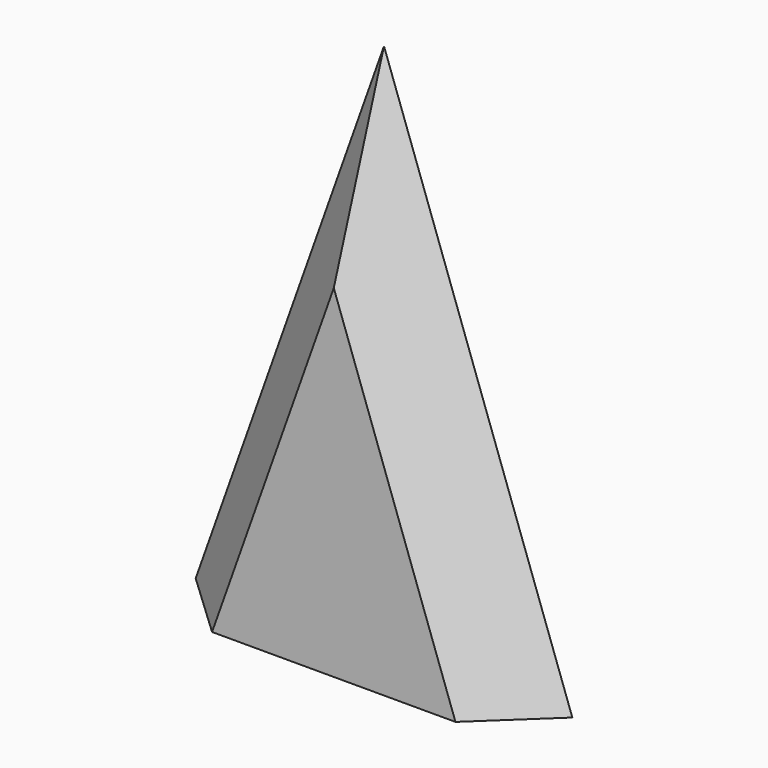
from build123d import *

# Parameters (mm, degrees)
F1_DEPTH      = 2.54
F1_DEPTH_BACK = 2.54
F2_R          = 1.905
F3_DEPTH      = 5.08
F4_SIZE       = 2.53999


# Not quite as in the source:
# - a fillet or chamfer is up to 0.001 mm smaller than in the source, because OpenCascade refuses the exact size


with BuildPart() as f1:
    # F0 (on Front) → F1 (new body, two sides)
    with BuildSketch(Plane.XZ) as f1_sk:
        Polygon((0, 21.4385549893), (-7.62, 0), (7.62, 0), align=None)
    extrude(amount=F1_DEPTH)
    extrude(f1_sk.sketch, amount=-F1_DEPTH_BACK)

    # F2 (on Top) → F3 (cut)
    with BuildSketch(Plane.XY):
        Circle(F2_R)
    extrude(amount=F3_DEPTH, mode=Mode.SUBTRACT)

    # F4 (size 2.54 in the source; OpenCascade refuses exactly that, so slightly less here)
    f4_edges = [f1.edges().sort_by_distance(p)[0] for p in [
        (3.81, -2.54, 10.719277),
        (-3.81, -2.54, 10.719277),
        (-3.81, 2.54, 10.719277),
        (3.81, 2.54, 10.719277),
    ]]
    chamfer(f4_edges, length=F4_SIZE)


solid = f1.part
